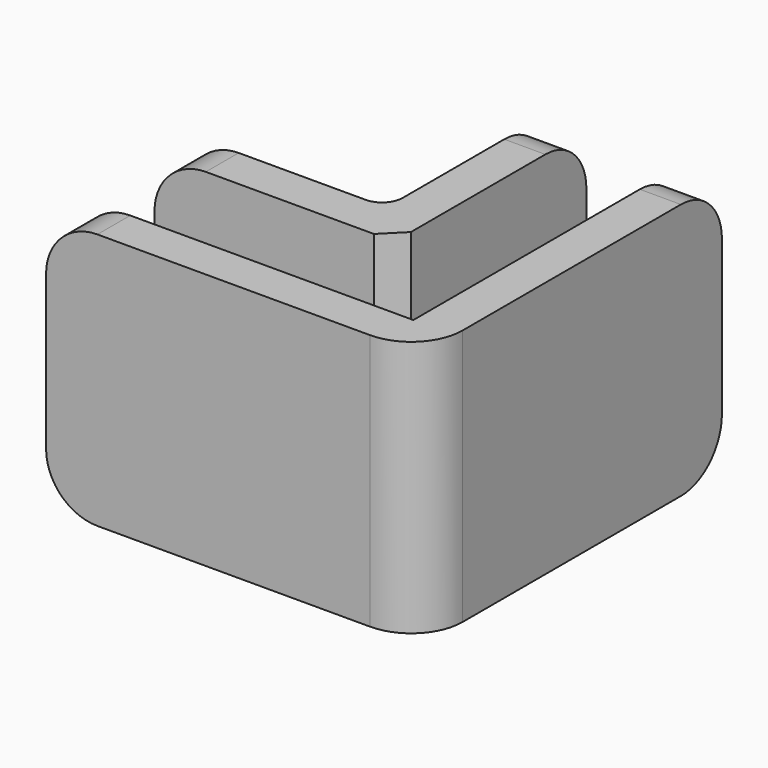
from build123d import *
from build123d import SkipClean  # not in build123d's __all__

# Parameters (mm, degrees)
F1_DEPTH       = 2
F2_DEPTH       = 25
F3_T1_DEPTH    = 29
F3_T3_DEPTH    = 29
F3_T5_DEPTH    = 29
F3_T7_DEPTH    = 29
F3_T9_DEPTH    = 42.2
F3_T11_DEPTH   = 42.2
F3_T13_DEPTH   = 50
F4_R           = 2
F5_SIZE        = 2
F7_D           = 3.3
F7_CSINK_D     = 6
F7_CSINK_ANGLE = 90


# Not quite as in the source:
# - a fillet or chamfer that OpenCascade refuses, or shapes differently, is made with other operations: its cross-section is extruded or revolved along the edge and cut away or added
# - a feature names something its author has since deleted; it is built from what else it names


with BuildPart() as f1:
    # F0 (on Top) → F1 (new body)
    with BuildSketch(Plane.XY):
        Polygon((4.9215265818, 0), (4.9215265818, 9.2), (4.9215265818, 32.5735770881), (-4.2784734182, 32.5735770881), (-4.2784734182, 9.2), (-27.6520505063, 9.2), (-27.6520505063, 0), (0, 0), align=None)
        Polygon((4.9215265818, 32.5735770881), (4.9215265818, 9.2), (4.9215265818, 0), (0, 0), (-27.6520505063, 0), (-27.6520505063, -4), (0, -4), (8.9215265818, -4), (8.9215265818, 32.5735770881), align=None)
        Polygon((-4.2784734182, 9.2), (-4.2784734182, 32.5735770881), (-8.2784734182, 32.5735770881), (-8.2784734182, 13.2), (-27.6520505063, 13.2), (-27.6520505063, 9.2), align=None)
    extrude(amount=F1_DEPTH)

    # F0 (on Top) → F2 (join)
    with BuildSketch(Plane.XY):
        Polygon((-4.2784734182, 9.2), (-4.2784734182, 32.5735770881), (-8.2784734182, 32.5735770881), (-8.2784734182, 13.2), (-27.6520505063, 13.2), (-27.6520505063, 9.2), align=None)
        Polygon((4.9215265818, 32.5735770881), (4.9215265818, 9.2), (4.9215265818, 0), (0, 0), (-27.6520505063, 0), (-27.6520505063, -4), (0, -4), (8.9215265818, -4), (8.9215265818, 32.5735770881), align=None)
    extrude(amount=F2_DEPTH)

    # F3: fillet of radius 5 on 7 edges, made by hand

    # F3_s2 → F3_t1 (cut)
    with BuildSketch(Plane.XZ.offset(-12.5)):
        with BuildLine():
            ThreePointArc((-22.6520505063, 25), (-26.1875844123, 23.5355339059), (-27.6520505063, 20))
            Line((-27.6520505063, 20), (-27.6520505063, 25))
            Line((-27.6520505063, 25), (-22.6520505063, 25))
        make_face()
    extrude(amount=F3_T1_DEPTH, mode=Mode.SUBTRACT)

    # F3_s4 → F3_t3 (cut)
    with BuildSketch(Plane.XZ.offset(-25.7)):
        with BuildLine():
            ThreePointArc((-22.6520505063, 25), (-26.1875844123, 23.5355339059), (-27.6520505063, 20))
            Line((-27.6520505063, 20), (-27.6520505063, 25))
            Line((-27.6520505063, 25), (-22.6520505063, 25))
        make_face()
    extrude(amount=F3_T3_DEPTH, mode=Mode.SUBTRACT)

    # F3_s6 → F3_t5 (cut)
    with BuildSketch(Plane.YZ.offset(-20.7784734182)):
        with BuildLine():
            ThreePointArc((27.5735770881, 25), (31.1091109941, 23.5355339059), (32.5735770881, 20))
            Line((32.5735770881, 20), (32.5735770881, 25))
            Line((32.5735770881, 25), (27.5735770881, 25))
        make_face()
    extrude(amount=F3_T5_DEPTH, mode=Mode.SUBTRACT)

    # F3_s8 → F3_t7 (cut)
    with BuildSketch(Plane.YZ.offset(-7.5784734182)):
        with BuildLine():
            ThreePointArc((32.5735770881, 20), (31.1091109941, 23.5355339059), (27.5735770881, 25))
            Line((27.5735770881, 25), (32.5735770881, 25))
            Line((32.5735770881, 25), (32.5735770881, 20))
        make_face()
    with SkipClean():  # cleaning this boolean's faces spoils the solid; the shape is the same uncleaned
        extrude(amount=F3_T7_DEPTH, mode=Mode.SUBTRACT)

    # F3_s10 → F3_t9 (cut)
    with BuildSketch(Plane.XZ.offset(-25.7)):
        with BuildLine():
            ThreePointArc((-22.6520505063, 0), (-26.1875844123, 1.4644660941), (-27.6520505063, 5))
            Line((-27.6520505063, 5), (-27.6520505063, 0))
            Line((-27.6520505063, 0), (-22.6520505063, 0))
        make_face()
    extrude(amount=F3_T9_DEPTH, mode=Mode.SUBTRACT)

    # F3_s12 → F3_t11 (cut)
    with BuildSketch(Plane.YZ.offset(-20.7784734182)):
        with BuildLine():
            ThreePointArc((27.5735770881, 0), (31.1091109941, 1.4644660941), (32.5735770881, 5))
            Line((32.5735770881, 5), (32.5735770881, 0))
            Line((32.5735770881, 0), (27.5735770881, 0))
        make_face()
    extrude(amount=F3_T11_DEPTH, mode=Mode.SUBTRACT)

    # F3_s14 → F3_t13 (cut)
    with BuildSketch(Plane.XY.offset(-12.5)):
        with BuildLine():
            ThreePointArc((3.9215265818, -4), (7.4570604877, -2.5355339059), (8.9215265818, 1))
            Line((8.9215265818, 1), (8.9215265818, -4))
            Line((8.9215265818, -4), (3.9215265818, -4))
        make_face()
    extrude(amount=F3_T13_DEPTH, mode=Mode.SUBTRACT)

    # F4
    f4_edges = [f1.edges().sort_by_distance(p)[0] for p in [
        (-8.278473, 13.2, 12.5),
    ]]
    fillet(f4_edges, radius=F4_R)

    # F5
    f5_edges = [f1.edges().sort_by_distance(p)[0] for p in [
        (-4.278473, 9.2, 13.5),
    ]]
    chamfer(f5_edges, length=F5_SIZE)

    # F7 (through all)
    with Locations(Plane(origin=(0, 0, 0), x_dir=(1, 0, 0), z_dir=(0, 0, -1))):
        with Locations((-15, -4.6), (0, -19.6)):
            CounterSinkHole(F7_D / 2, F7_CSINK_D / 2, counter_sink_angle=F7_CSINK_ANGLE)


solid = f1.part
